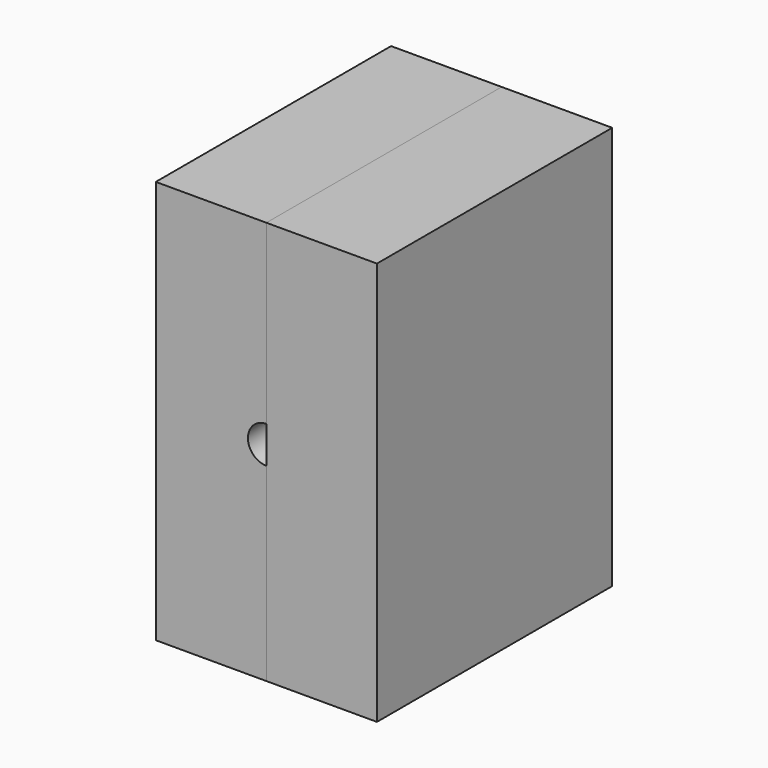
from build123d import *

# Parameters (mm, degrees)
F2_W     = 20.2671834268
F2_H     = 27.8065428138
F3_DEPTH = 7.62
F4_DEPTH = 7.62
F7_DEPTH = 4.445


# Not quite as in the source:
# - after a boolean that leaves OpenCascade's solid faulty, fix() repairs it


with BuildPart() as f1:
    # F0 (on Top) → F1 (revolve)
    with BuildSketch(Plane.XY):
        with BuildLine():
            Line((0, 12.7), (0, 0))
            ThreePointArc((0, 0), (6.35, 6.35), (0, 12.7))
        make_face()
    revolve(axis=Axis((0, 6.35, 0), (0, 1, 0)))


with BuildPart() as f3:
    # F2 (on Right) → F3 (new body)
    with BuildSketch(Plane.YZ):
        with Locations((5.7474102359, -0.4277937114)):
            Rectangle(F2_W, F2_H)
    extrude(amount=F3_DEPTH)

    # F5: cut F1
    add(f1.part, mode=Mode.SUBTRACT)

    add(f3.part.fix(), mode=Mode.REPLACE)


with BuildPart() as f4:
    # F2 (on Right) → F4 (new body)
    with BuildSketch(Plane.YZ):
        with Locations((5.7474102359, -0.4277937114)):
            Rectangle(F2_W, F2_H)
    extrude(amount=-F4_DEPTH)

    # F5: cut F1
    add(f1.part, mode=Mode.SUBTRACT)

    # F6 (on face) → F7 (cut)
    with BuildSketch(Plane.XZ.offset(4.3861814775)):
        with BuildLine():
            ThreePointArc((0, 1.27), (-1.27, 0), (0, -1.27))
            Line((0, -1.27), (0, 1.27))
        make_face()
    extrude(amount=-F7_DEPTH, mode=Mode.SUBTRACT)


solid = Compound([f3.part, f4.part])
